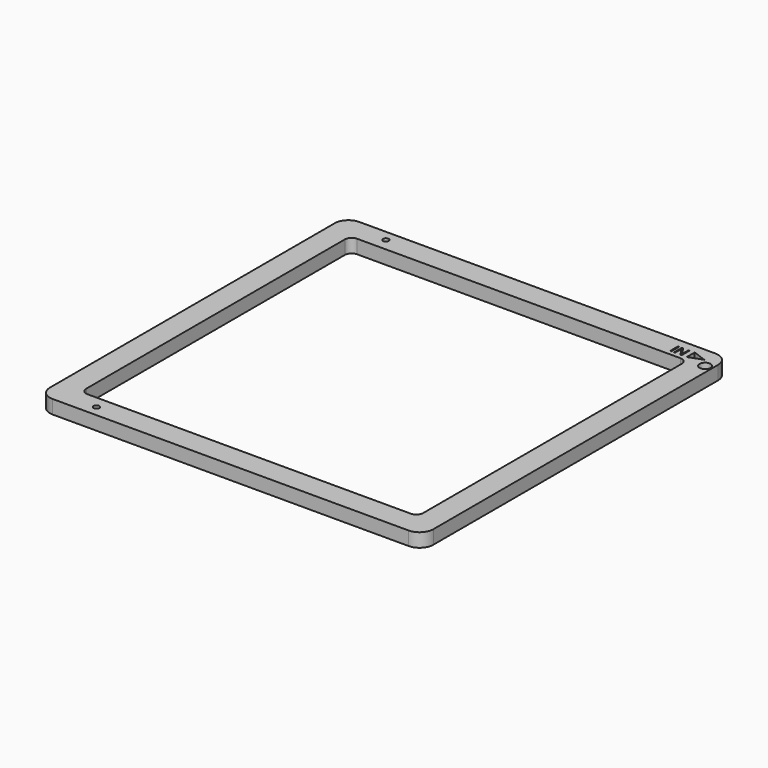
from build123d import *

# Parameters (mm, degrees)
F1_DEPTH     = 10
F2_R         = 2.1
F2_R_2       = 4
F3_DEPTH     = 4.5
F4_TEXT_SIZE = 10.1102842852
F5_DEPTH     = 10.001


# Not quite as in the source:
# - Text() gives the source's letters only with a copy of the font that has no kerning and outlines rounded to 1/6400 em; it was checked with that copy


with BuildPart() as f1:
    # F0 (on Top) → F1 (new body)
    with BuildSketch(Plane.XY):
        with BuildLine():
            ThreePointArc((140, 130), (137.0710678119, 137.0710678119), (130, 140))
            Line((130, 140), (-130, 140))
            ThreePointArc((-130, 140), (-137.0710678119, 137.0710678119), (-140, 130))
            Line((-140, 130), (-140, -130))
            ThreePointArc((-140, -130), (-137.0710678119, -137.0710678119), (-130, -140))
            Line((-130, -140), (130, -140))
            ThreePointArc((130, -140), (137.0710678119, -137.0710678119), (140, -130))
            Line((140, -130), (140, 130))
        make_face()
    extrude(amount=F1_DEPTH)

    # F2 (on face) → F3 (cut)
    with BuildSketch(Plane.XY.offset(10)):
        with Locations((-104.3, 132.15)):
            Circle(F2_R)
        with Locations((135, 124.35)):
            Circle(F2_R_2)
        with Locations((-104.3, -132.15)):
            Circle(F2_R)
    extrude(amount=-F3_DEPTH, mode=Mode.SUBTRACT)

    # F4 (on face) + F1_face1 (on face) → F5 (cut, through all)
    with BuildSketch(Plane.XY.offset(10)):
        Polygon((120, 126.3602976573), (130, 130), (120, 133.6397023427), align=None)
        with BuildLine():
            Line((118, 123), (-118, 123))
            ThreePointArc((-118, 123), (-121.5355339059, 121.5355339059), (-123, 118))
            Line((-123, 118), (-123, -118))
            ThreePointArc((-123, -118), (-121.5355339059, -121.5355339059), (-118, -123))
            Line((-118, -123), (118, -123))
            ThreePointArc((118, -123), (121.5355339059, -121.5355339059), (123, -118))
            Line((123, -118), (123, 118))
            ThreePointArc((123, 118), (121.5355339059, 121.5355339059), (118, 123))
        make_face()
        with Locations((106.8960346425, 126.3602976573)):
            Text('IN', F4_TEXT_SIZE, font='Open Sans', text_align=(TextAlign.LEFT, TextAlign.BOTTOM))
    with BuildSketch(Plane(origin=(0, 0, 0), x_dir=(1, 0, 0), z_dir=(0, 0, -1))):
        with BuildLine():
            ThreePointArc((130, -140), (137.0710678119, -137.0710678119), (140, -130))
            Line((140, -130), (140, 130))
            ThreePointArc((140, 130), (137.0710678119, 137.0710678119), (130, 140))
            Line((130, 140), (-130, 140))
            ThreePointArc((-130, 140), (-137.0710678119, 137.0710678119), (-140, 130))
            Line((-140, 130), (-140, -130))
            ThreePointArc((-140, -130), (-137.0710678119, -137.0710678119), (-130, -140))
            Line((-130, -140), (130, -140))
        make_face()
    extrude(amount=-F5_DEPTH, dir=(0, 0, 1), mode=Mode.SUBTRACT)


solid = f1.part
